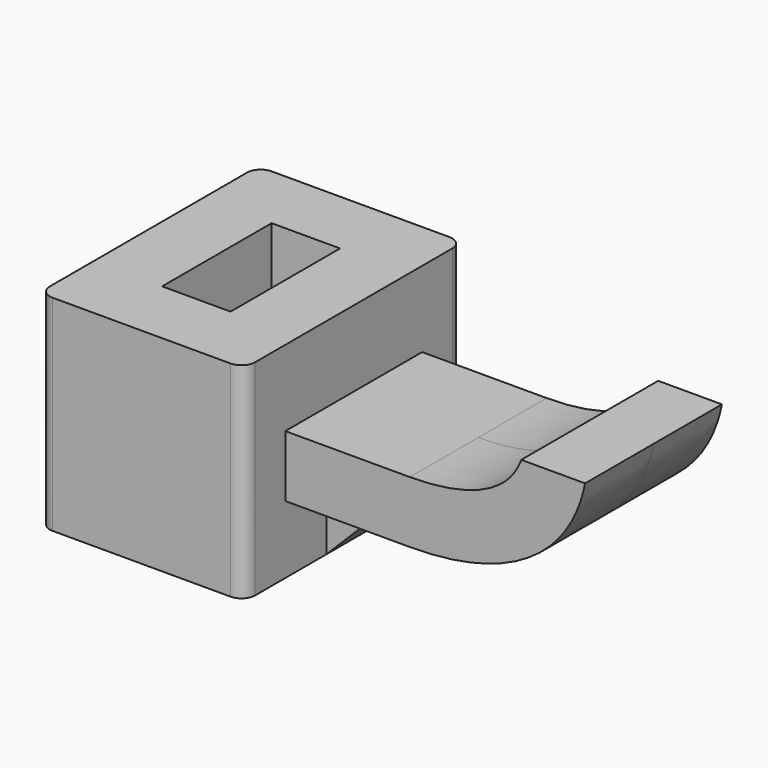
from build123d import *

# Parameters (mm, degrees)
F1_DEPTH     = 20
F2_DEPTH     = 12.5
F3_DEPTH     = 5
F4_R         = 2
F5_T         = 10
F5_T3_DEPTH  = 29.9026188965
F5_T5_DEPTH  = 27.5
F5_T7_DEPTH  = 27.5
F5_T9_DEPTH  = 29
F5_T11_DEPTH = 45
F5_T13_DEPTH = 29.9026188965
F5_T15_DEPTH = 30


# Not quite as in the source:
# - ends of sketch curves that miss each other by under 0.0002 mm in the source are joined
# - a shell that OpenCascade refuses in one call is made with other operations: the cavity is built on its own and cut out


with BuildPart() as f1:
    # F0 (on Front) → F1 (new body, symmetric)
    with BuildSketch(Plane.XZ):
        Polygon((-98.8679975982, 54.1129348578), (-128.8679975982, 54.1129348578), (-128.8679975982, 24.1129348578), (-98.8679975982, 24.1129348578), (-98.8679975982, 34.0155537543), (-98.8679975982, 43.0155537543), align=None)
    extrude(amount=F1_DEPTH, both=True)

    # F0 (on Front) → F2 (join, symmetric)
    with BuildSketch(Plane.XZ):
        with BuildLine():
            Line((-80.6820849815, 43.0155537543), (-98.8679975982, 43.0155537543))
            Line((-98.8679975982, 43.0155537543), (-98.8679975982, 34.0155537543))
            Line((-98.8679975982, 34.0155537543), (-88.9653787017, 34.0155537543))
            Line((-88.9653787017, 34.0155537543), (-80.682094855, 34.0155537543))
            add(Edge.make_bspline(
                [(-80.682094855, 34.0155537543), (-66.1309954288, 34.0155509655), (-57.1216260093, 40.1806794107), (-55.0665845173, 50.5349263549)],
                knots=[0, 0, 0, 0, 30.4802237684, 30.4802237684, 30.4802237684, 30.4802237684], degree=3))
            Line((-55.0665845173, 50.5349263549), (-64.3839240074, 50.5349263549))
            add(Edge.make_bspline(
                [(-80.6820849815, 43.0155537543), (-79.1809668737, 43.0155537553), (-76.3999490421, 43.1750788515), (-72.9213473732, 43.8149397212), (-70.1430488739, 44.758463036), (-68.0271542887, 45.9005167962), (-66.4709613794, 47.1632066722), (-65.3230275472, 48.5510213805), (-64.6991129712, 49.71943479), (-64.4207731634, 50.4356187157), (-64.3839240074, 50.5349263549)],
                knots=[2.262e-07, 2.262e-07, 2.262e-07, 2.262e-07, 0.125, 0.25, 0.375, 0.5, 0.625, 0.75, 0.875, 0.8947169283, 0.8947169283, 0.8947169283, 0.8947169283], degree=3))
        make_face()
    extrude(amount=F2_DEPTH, both=True)

    # F0 (on Front) → F3 (join, symmetric)
    with BuildSketch(Plane.XZ):
        Polygon((-98.8679975982, 34.0155537543), (-98.8679975982, 24.1129348578), (-88.9653787017, 34.0155537543), align=None)
    extrude(amount=F3_DEPTH, both=True)

    # F4
    f4_edges = [f1.edges().sort_by_distance(p)[0] for p in [
        (-98.867998, -20, 39.112935),
        (-128.867998, -20, 39.112935),
        (-98.867998, 20, 39.112935),
        (-128.867998, 20, 39.112935),
    ]]
    fillet(f4_edges, radius=F4_R)

    # F5: shell of thickness 10, made by hand


with BuildPart() as f5_core1:
    # F5_t2: copy of F1
    add(f1.part)

    # the walls: a layer under each face that stays
    f5_faces = [f5_core1.faces().sort_by_distance(p)[0] for p in [
        (-113.8679975982, 20, 39.1129348578),
        (-98.8679975982, 12, 29.1129348578),
        (-128.8679975982, 0, 39.1129348578),
        (-113.8679975982, -20, 39.1129348578),
        (-113.8679975982, 0, 24.1129348578),
        (-97.2175611154, -5, 29.0642443061),
        (-97.2175611154, 5, 29.0642443061),
        (-95.8370138076, 8.3333333333, 34.0155537543),
        (-76.9672910577, -12.5, 42.2752386602),
        (-76.9672910577, 12.5, 42.2752386602),
        (-89.7750412898, 0, 43.0155537543),
        (-93.9166881499, 0, 29.0642443061),
        (-63.1883179608, -6.25, 38.3923964047),
        (-63.1883179608, 6.25, 38.3923964047),
        (-59.7252542624, 0, 50.5349263549),
        (-68.9445639905, -6.25, 45.4259334498),
        (-68.9445639905, 6.25, 45.4259334498),
    ]]
    thicken(f5_faces, amount=-F5_T, mode=Mode.SUBTRACT)

    # F5_s4 → F5_t3 (cut)
    with BuildSketch(Plane.XY.offset(14.1129348578)):
        Polygon((-98.7679975982, -5.1), (-108.8679975982, -5), (-108.8679975982, 5), (-98.8679975982, 5), align=None)
        Polygon((-98.7679975982, 5.1), (-108.8679975982, 5), (-108.8679975982, -5), (-98.8679975982, -5), align=None)
    extrude(amount=F5_T3_DEPTH, mode=Mode.SUBTRACT)

    # F5_s6 → F5_t5 (cut)
    with BuildSketch(Plane.XZ.offset(-5)):
        Polygon((-98.7679975982, 33.9155537543), (-108.8679975982, 34.0155537543), (-108.8679975982, 44.0155537543), (-98.8679975982, 44.0155537543), align=None)
    extrude(amount=F5_T5_DEPTH, mode=Mode.SUBTRACT)

    # F5_s8 → F5_t7 (cut)
    with BuildSketch(Plane.XZ.offset(-22.5)):
        Polygon((-98.7679975982, 33.9155537543), (-108.8679975982, 34.0155537543), (-108.8679975982, 44.0155537543), (-98.8679975982, 44.0155537543), align=None)
    extrude(amount=F5_T7_DEPTH, mode=Mode.SUBTRACT)

    # F5_s10 → F5_t9 (cut)
    with BuildSketch(Plane.XY.offset(24.0155537543)):
        Polygon((-98.7679975982, -12.6), (-108.8679975982, -12.5), (-108.8679975982, -2.5), (-98.8679975982, -2.5), align=None)
        Polygon((-98.7679975982, 12.6), (-108.8679975982, 12.5), (-108.8679975982, 2.5), (-98.8679975982, 2.5), align=None)
    extrude(amount=F5_T9_DEPTH, mode=Mode.SUBTRACT)

    # F5_s12 → F5_t11 (cut)
    with BuildSketch(Plane.XZ.offset(-22.5)):
        Polygon((-98.7679975982, 43.1155537543), (-108.8679975982, 43.0155537543), (-108.8679975982, 33.0155537543), (-98.8679975982, 33.0155537543), align=None)
    extrude(amount=F5_T11_DEPTH, mode=Mode.SUBTRACT)

    # F5_s14 → F5_t13 (cut)
    with BuildSketch(Plane.YZ.offset(-108.8679975982)):
        Polygon((-5.1, 33.9155537543), (5, 34.0155537543), (5, 44.0155537543), (-5, 44.0155537543), align=None)
        Polygon((5.1, 33.9155537543), (-5, 34.0155537543), (-5, 44.0155537543), (5, 44.0155537543), align=None)
    extrude(amount=F5_T13_DEPTH, mode=Mode.SUBTRACT)

    # F5_s16 → F5_t15 (cut)
    with BuildSketch(Plane.XZ.offset(-15)):
        Polygon((-88.8946680236, 33.8448430762), (-88.9653787017, 44.0155537543), (-93.1075143254, 44.0155537543), (-96.0364465136, 41.0866215662), align=None)
    extrude(amount=F5_T15_DEPTH, mode=Mode.SUBTRACT)


with BuildPart() as f1_1:
    add(f1.part)

    # what is left inside the walls is the cavity
    f5_cavity = [f5_core1.part.solids().sort_by_distance(p)[0] for p in [
        (-118.767998, 3.333333, 44.112935),
    ]]
    add(f5_cavity, mode=Mode.SUBTRACT)


solid = f1_1.part
